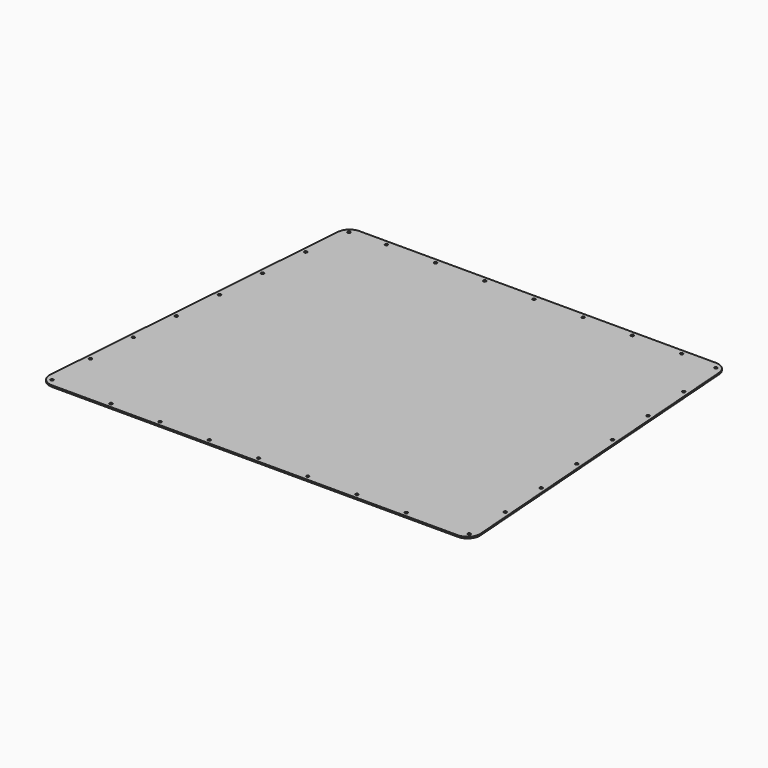
from build123d import *

# Parameters (mm, degrees)
F1_DEPTH = 1.5748
F3_D     = 2.9464


# Not quite as in the source:
# - a feature names something its author has since deleted; it is built from what else it names


with BuildPart() as f1:
    # F0 (on Top) → F1 (new body)
    with BuildSketch(Plane.XY):
        with BuildLine():
            Line((53.975, 352.425), (-53.975, 352.425))
            Line((-53.975, 352.425), (-184.15, 352.425))
            ThreePointArc((-184.15, 352.425), (-192.7889958635, 349.0340144736), (-196.8146515797, 340.6718898377))
            Line((-196.8146515797, 340.6718898377), (-222.2146515797, 0.9468898377))
            ThreePointArc((-222.2146515797, 0.9468898377), (-218.8590144736, -8.6389958635), (-209.55, -12.7))
            Line((-209.55, -12.7), (-53.975, -12.7))
            Line((-53.975, -12.7), (53.975, -12.7))
            Line((53.975, -12.7), (209.55, -12.7))
            ThreePointArc((209.55, -12.7), (218.8590144736, -8.6389958635), (222.2146515797, 0.9468898377))
            Line((222.2146515797, 0.9468898377), (196.8146515797, 340.6718898377))
            ThreePointArc((196.8146515797, 340.6718898377), (192.7889958635, 349.0340144736), (184.15, 352.425))
            Line((184.15, 352.425), (53.975, 352.425))
        make_face()
    extrude(amount=F1_DEPTH)

    # F3 (through all)
    with Locations(Plane.XY.offset(1.5748)):
        with Locations((-152.4, 347.6625), (-101.6, 347.6625), (-50.8, 347.6625), (0, 347.6625), (50.8, 347.6625), (101.6, 347.6625), (152.4, 347.6625), (195.3143273232, 296.8625), (199.1124581643, 246.0625), (202.9105890054, 195.2625), (206.7087198466, 144.4625), (210.5068506877, 93.6625), (214.3049815288, 42.8625), (152.4, -7.9375), (101.6, -7.9375), (50.8, -7.9375), (0, -7.9375), (-50.8, -7.9375), (-101.6, -7.9375), (-152.4, -7.9375), (-214.3049815288, 42.8625), (-210.5068506877, 93.6625), (-206.7087198466, 144.4625), (-202.9105890054, 195.2625), (-199.1124581643, 246.0625), (-195.3143273232, 296.8625), (215.368134046, -5.3993724147), (-215.368134046, -5.3993724147), (-189.5493724147, 345.543134046), (189.5493724147, 345.543134046)):
            Hole(F3_D / 2)


with BuildPart() as f4_1:
    # F4: instance of F1
    add(f1.part.mirror(Plane.YZ))


solid = Compound([f1.part, f4_1.part])
